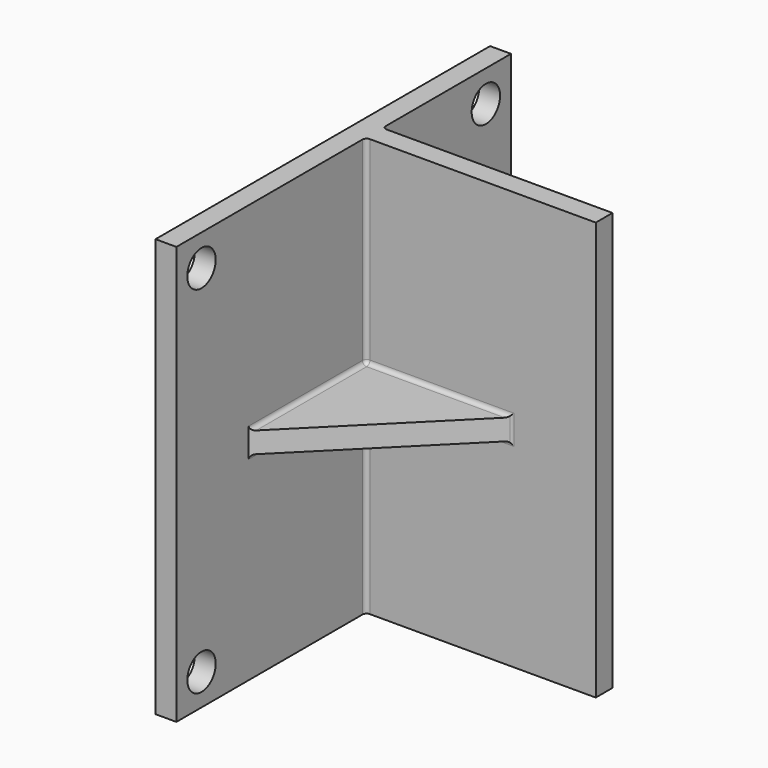
from build123d import *

# Parameters (mm, degrees)
F1_DEPTH = 200
F2_R     = 8.5
F3_DEPTH = 10.001
F4_W     = 70
F4_H     = 10
F5_DEPTH = 70
F7_DEPTH = 10
F8_R     = 2


with BuildPart() as f1:
    # F0 (on Top) → F1 (new body)
    with BuildSketch(Plane.XY):
        Polygon((-12.944079712, 104.5888163149), (-22.944079712, 104.5888163149), (-22.944079712, -95.4111836851), (-12.944079712, -95.4111836851), (-12.944079712, 17.7888163149), (97.055920288, 17.7888163149), (97.055920288, 27.7888163149), (-12.944079712, 27.7888163149), align=None)
    extrude(amount=F1_DEPTH)

    # F2 (on face) → F3 (cut, through all)
    with BuildSketch(Plane.YZ.offset(-12.944079712)):
        with Locations((89.5888163149, 185)):
            Circle(F2_R)
        with Locations((89.5888163149, 15)):
            Circle(F2_R)
        with Locations((-80.4111836851, 15)):
            Circle(F2_R)
        with Locations((-80.4111836851, 185)):
            Circle(F2_R)
    extrude(amount=-F3_DEPTH, mode=Mode.SUBTRACT)

    # F4 (on face) → F5 (join)
    with BuildSketch(Plane.YZ.offset(-12.944079712)):
        with Locations((-17.2111836851, 100)):
            Rectangle(F4_W, F4_H)
    extrude(amount=F5_DEPTH)

    # F6 (on face) → F7 (cut)
    with BuildSketch(Plane.XY.offset(105)):
        Polygon((57.055920288, 17.7888163149), (-12.944079712, -52.2111836851), (57.055920288, -52.2111836851), align=None)
    extrude(amount=-F7_DEPTH, mode=Mode.SUBTRACT)

    # F8
    f8_edges = [f1.edges().sort_by_distance(p)[0] for p in [
        (-12.94408, 17.788816, 152.5),
        (-12.94408, -17.211184, 105),
        (-12.94408, -17.211184, 95),
        (-12.94408, 17.788816, 47.5),
        (-12.94408, 27.788816, 100),
        (57.05592, 17.788816, 100),
        (22.05592, 17.788816, 105),
        (22.05592, 17.788816, 95),
    ]]
    fillet(f8_edges, radius=F8_R)


solid = f1.part
